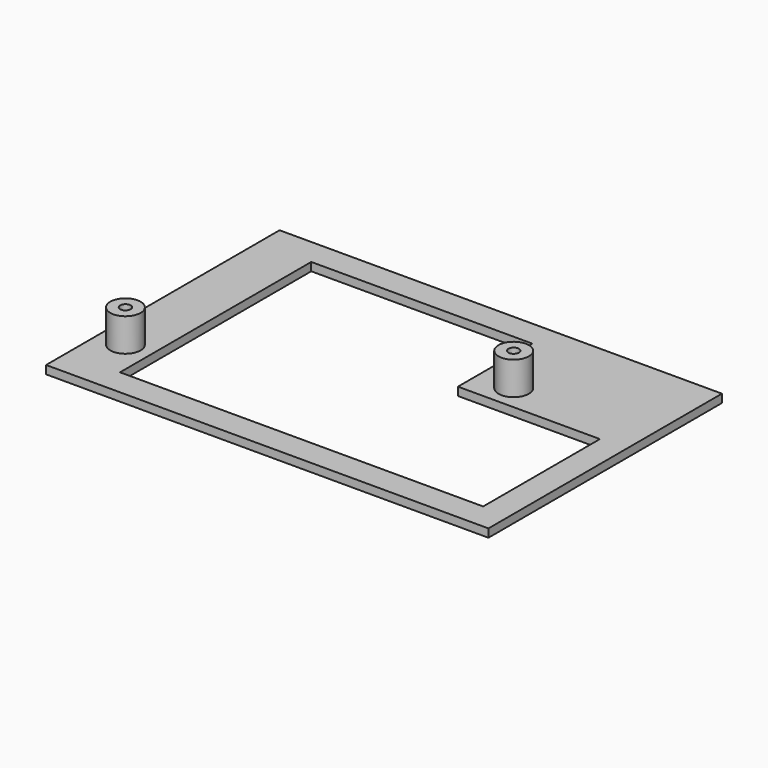
from build123d import *

# Parameters (mm, degrees)
F0_W     = 85.09
F0_H     = 56.134
F1_DEPTH = 1.5875
F2_R     = 2.921
F2_R_2   = 1.016
F3_DEPTH = 6.35
F4_DEPTH = 6.35
F5_W     = 32.385
F5_H     = 22.987
F5_W_2   = 27.305
F5_H_2   = 5.08
F6_DEPTH = 6.35


# Not quite as in the source:
# - a feature names something its author has since deleted; it is built from what else it names


with BuildPart() as f1:
    # F0 (on Top) → F1 (new body)
    with BuildSketch(Plane.XY):
        Rectangle(F0_W, F0_H)
    extrude(amount=F1_DEPTH)

    # F2 (on face) → F3 (join)
    with BuildSketch(Plane.XY.offset(1.5875)):
        with Locations((17.018, 9.906)):
            Circle(F2_R)
        with Locations((17.018, 9.906)):
            Circle(F2_R_2, mode=Mode.SUBTRACT)
        with Locations((-37.338, -15.494)):
            Circle(F2_R)
        with Locations((-37.338, -15.494)):
            Circle(F2_R_2, mode=Mode.SUBTRACT)
    extrude(amount=F3_DEPTH)

    # F2 (on face) → F4 (cut)
    with BuildSketch(Plane.XY.offset(1.5875)):
        with Locations((-37.338, -15.494)):
            Circle(F2_R_2)
        with Locations((17.018, 9.906)):
            Circle(F2_R_2)
    extrude(amount=-F4_DEPTH, mode=Mode.SUBTRACT)

    # F5 (on face) → F6 (cut)
    with BuildSketch(Plane.XY.offset(1.5875)):
        with Locations((-16.1925, 11.4935)):
            Rectangle(F5_W, F5_H)
        Polygon((0, 22.987), (0, 0), (10.16, 0), (10.16, 5.08), (10.16, 22.987), align=None)
        with Locations((23.8125, 2.54)):
            Rectangle(F5_W_2, F5_H_2)
        Polygon((10.16, 0), (0, 0), (0, -22.987), (37.465, -22.987), (37.465, 0), align=None)
        with Locations((-16.1925, -11.4935)):
            Rectangle(F5_W, F5_H)
    extrude(amount=-F6_DEPTH, mode=Mode.SUBTRACT)


solid = f1.part
